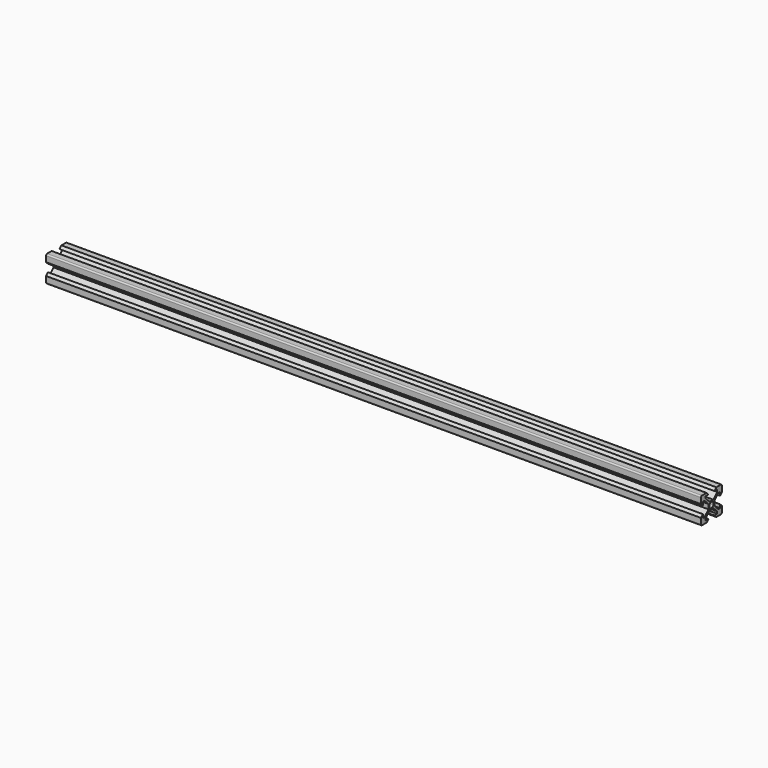
from build123d import *

# Parameters (mm, degrees)
F1_DEPTH = 500


# Not quite as in the source:
# - ends of sketch curves that miss each other by under 0.0002 mm in the source are joined


with BuildPart() as f1:
    # F0 (on Right) → F1 (new body)
    with BuildSketch(Plane.YZ):
        with BuildLine():
            Line((8.2, -10), (9, -10))
            ThreePointArc((9, -10), (9.7071067812, -9.7071067812), (10, -9))
            Line((10, -9), (10, -8.2))
            Line((10, -8.2), (8.2, -8.2))
            Line((8.2, -8.2), (8.2, -10))
        make_face()
        Polygon((5.4993398282, -8.2), (7.1393398282, -8.2), (5.4993398282, -6.56), align=None)
        Polygon((6.56, -5.4993398282), (8.2, -7.1393398282), (8.2, -5.4993398282), align=None)
        with BuildLine():
            Line((8.2, 10), (8.2, 8.2))
            Line((8.2, 8.2), (10, 8.2))
            Line((10, 8.2), (10, 9))
            ThreePointArc((10, 9), (9.7071067812, 9.7071067812), (9, 10))
            Line((9, 10), (8.2, 10))
        make_face()
        Polygon((8.2, 7.1393398282), (6.56, 5.4993398282), (8.2, 5.4993398282), align=None)
        Polygon((5.4993398282, 8.2), (5.4993398282, 6.56), (7.1393398282, 8.2), align=None)
        with BuildLine():
            Line((-9.9999004684, 8.2000055944), (-8.1999004684, 8.2000055944))
            Line((-8.1999004684, 8.2000055944), (-8.1999004684, 10.0000055944))
            Line((-8.1999004684, 10.0000055944), (-8.9999004684, 10.0000055944))
            ThreePointArc((-8.9999004684, 10.0000055944), (-9.7070072496, 9.7071123756), (-9.9999004684, 9.0000055944))
            Line((-9.9999004684, 9.0000055944), (-9.9999004684, 8.2000055944))
        make_face()
        Polygon((-7.1392402967, 8.2000055944), (-5.4992402967, 6.5600055944), (-5.4992402967, 8.2000055944), align=None)
        Polygon((-8.1999004684, 5.4993454226), (-6.5599004684, 5.4993454226), (-8.1999004684, 7.1393454226), align=None)
        with BuildLine():
            Line((-8.1999004684, -9.9999944056), (-8.1999004684, -8.1999944056))
            Line((-8.1999004684, -8.1999944056), (-9.9999004684, -8.1999944056))
            Line((-9.9999004684, -8.1999944056), (-9.9999004684, -8.9999944056))
            ThreePointArc((-9.9999004684, -8.9999944056), (-9.7070072496, -9.7071011868), (-8.9999004684, -9.9999944056))
            Line((-8.9999004684, -9.9999944056), (-8.1999004684, -9.9999944056))
        make_face()
        Polygon((-8.1999004684, -7.1393342338), (-6.5599004684, -5.4993342338), (-8.1999004684, -5.4993342338), align=None)
        Polygon((-5.4992402967, -8.1999944056), (-5.4992402967, -6.5599944056), (-7.1392402967, -8.1999944056), align=None)
        with BuildLine():
            Line((1.9173232366, -0.8566630648), (2.84, -1.7793398282))
            Line((2.84, -1.7793398282), (2.84, 0))
            Line((2.84, 0), (2.1, 0))
            ThreePointArc((2.1, 0), (2.0538231176, -0.4379618723), (1.9173232366, -0.8566630648))
        make_face()
        with BuildLine():
            Line((0, -2.84), (1.7793398282, -2.84))
            Line((1.7793398282, -2.84), (0.8566630648, -1.9173232366))
            ThreePointArc((0.8566630648, -1.9173232366), (0.4379618723, -2.0538231176), (0, -2.1))
            Line((0, -2.1), (0, -2.84))
        make_face()
        with BuildLine():
            Line((-1.7792402967, -2.8399944056), (9.95316e-05, -2.8399944056))
            Line((9.95316e-05, -2.8399944056), (0, -2.1))
            ThreePointArc((0, -2.1), (-0.4378623408, -2.0538175232), (-0.8565635332, -1.9173176422))
            Line((-0.8565635332, -1.9173176422), (-1.7792402967, -2.8399944056))
        make_face()
        Polygon((4.64, -10), (8.2, -10), (8.2, -8.2), (7.1393398282, -8.2), (5.4993398282, -8.2), (2.84, -8.2), align=None)
        Polygon((8.2, -8.2), (10, -8.2), (10, -4.64), (8.2, -2.84), (8.2, -5.4993398282), (8.2, -7.1393398282), align=None)
        with BuildLine():
            ThreePointArc((0, 2.1), (0.4379618723, 2.0538231176), (0.8566630648, 1.9173232366))
            Line((0.8566630648, 1.9173232366), (1.7793398282, 2.84))
            Line((1.7793398282, 2.84), (0, 2.84))
            Line((0, 2.84), (0, 2.1))
        make_face()
        with BuildLine():
            Line((2.1, 0), (2.84, 0))
            Line((2.84, 0), (2.84, 1.7793398282))
            Line((2.84, 1.7793398282), (1.9173232366, 0.8566630648))
            ThreePointArc((1.9173232366, 0.8566630648), (2.0538231176, 0.4379618723), (2.1, 0))
        make_face()
        with BuildLine():
            ThreePointArc((-0.8565635332, 1.917328831), (-0.4378623408, 2.053828712), (9.95316e-05, 2.1000055944))
            Line((9.95316e-05, 2.1000055944), (0, 2.84))
            Line((0, 2.84), (-1.7792402967, 2.8400055944))
            Line((-1.7792402967, 2.8400055944), (-0.8565635332, 1.917328831))
        make_face()
        Polygon((8.2, 8.2), (8.2, 7.1393398282), (8.2, 5.4993398282), (8.2, 2.84), (10, 4.64), (10, 8.2), align=None)
        Polygon((7.1393398282, 8.2), (8.2, 8.2), (8.2, 10), (4.64, 10), (2.84, 8.2), (5.4993398282, 8.2), align=None)
        with BuildLine():
            Line((-2.8399004684, 1.7793454226), (-2.8399004684, 5.5944e-06))
            Line((-2.8399004684, 5.5944e-06), (-2.0999004684, 5.5944e-06))
            ThreePointArc((-2.0999004684, 5.5944e-06), (-2.053723586, 0.4379674667), (-1.917223705, 0.8566686592))
            Line((-1.917223705, 0.8566686592), (-2.8399004684, 1.7793454226))
        make_face()
        Polygon((-8.1999004684, 10.0000055944), (-8.1999004684, 8.2000055944), (-7.1392402967, 8.2000055944), (-5.4992402967, 8.2000055944), (-2.8399004684, 8.2000055944), (-4.6399004684, 10.0000055944), align=None)
        Polygon((-8.1999004684, 5.4993454226), (-8.1999004684, 7.1393454226), (-8.1999004684, 8.2000055944), (-9.9999004684, 8.2000055944), (-9.9999004684, 4.6400055944), (-8.1999004684, 2.8400055944), align=None)
        with BuildLine():
            Line((-2.8399004684, 5.5944e-06), (-2.8399004684, -1.7793342338))
            Line((-2.8399004684, -1.7793342338), (-1.917223705, -0.8566574704))
            ThreePointArc((-1.917223705, -0.8566574704), (-2.053723586, -0.4379562779), (-2.0999004684, 5.5944e-06))
            Line((-2.0999004684, 5.5944e-06), (-2.8399004684, 5.5944e-06))
        make_face()
        Polygon((-9.9999004684, -8.1999944056), (-8.1999004684, -8.1999944056), (-8.1999004684, -7.1393342338), (-8.1999004684, -5.4993342338), (-8.1999004684, -2.8399944056), (-9.9999004684, -4.6399944056), align=None)
        Polygon((-5.4992402967, -8.1999944056), (-7.1392402967, -8.1999944056), (-8.1999004684, -8.1999944056), (-8.1999004684, -9.9999944056), (-4.6399004684, -9.9999944056), (-2.8399004684, -8.1999944056), align=None)
        with BuildLine():
            Line((-2.8399004684, -1.7793342338), (-1.7792402967, -2.8399944056))
            Line((-1.7792402967, -2.8399944056), (-0.8565635332, -1.9173176422))
            ThreePointArc((-0.8565635332, -1.9173176422), (-1.4848247089, -1.4849186461), (-1.917223705, -0.8566574704))
            Line((-1.917223705, -0.8566574704), (-2.8399004684, -1.7793342338))
        make_face()
        Polygon((-4.4695703825, -5.5303244915), (-1.7792402967, -2.8399944056), (-2.8399004684, -1.7793342338), (-5.5302305543, -4.4696643197), (-6.5599004684, -5.4993342338), (-8.1999004684, -7.1393342338), (-8.1999004684, -8.1999944056), (-7.1392402967, -8.1999944056), (-5.4992402967, -6.5599944056), align=None)
        with BuildLine():
            Line((7.1393398282, -8.2), (8.2, -8.2))
            Line((8.2, -8.2), (8.2, -7.1393398282))
            Line((8.2, -7.1393398282), (6.56, -5.4993398282))
            Line((6.56, -5.4993398282), (5.5303300859, -4.4696699141))
            Line((5.5303300859, -4.4696699141), (2.84, -1.7793398282))
            Line((2.84, -1.7793398282), (1.9173232366, -0.8566630648))
            ThreePointArc((1.9173232366, -0.8566630648), (1.4849242405, -1.4849242405), (0.8566630648, -1.9173232366))
            Line((0.8566630648, -1.9173232366), (1.7793398282, -2.84))
            Line((1.7793398282, -2.84), (4.4696699141, -5.5303300859))
            Line((4.4696699141, -5.5303300859), (5.4993398282, -6.56))
            Line((5.4993398282, -6.56), (7.1393398282, -8.2))
        make_face()
        with BuildLine():
            Line((1.9173232366, 0.8566630648), (2.84, 1.7793398282))
            Line((2.84, 1.7793398282), (5.5303300859, 4.4696699141))
            Line((5.5303300859, 4.4696699141), (6.56, 5.4993398282))
            Line((6.56, 5.4993398282), (8.2, 7.1393398282))
            Line((8.2, 7.1393398282), (8.2, 8.2))
            Line((8.2, 8.2), (7.1393398282, 8.2))
            Line((7.1393398282, 8.2), (5.4993398282, 6.56))
            Line((5.4993398282, 6.56), (4.4696699141, 5.5303300859))
            Line((4.4696699141, 5.5303300859), (1.7793398282, 2.84))
            Line((1.7793398282, 2.84), (0.8566630648, 1.9173232366))
            ThreePointArc((0.8566630648, 1.9173232366), (1.4849242405, 1.4849242405), (1.9173232366, 0.8566630648))
        make_face()
        with BuildLine():
            Line((-5.5302305543, 4.4696755085), (-2.8399004684, 1.7793454226))
            Line((-2.8399004684, 1.7793454226), (-1.917223705, 0.8566686592))
            ThreePointArc((-1.917223705, 0.8566686592), (-1.4848247089, 1.4849298349), (-0.8565635332, 1.917328831))
            Line((-0.8565635332, 1.917328831), (-1.7792402967, 2.8400055944))
            Line((-1.7792402967, 2.8400055944), (-4.4695703825, 5.5303356803))
            Line((-4.4695703825, 5.5303356803), (-5.4992402967, 6.5600055944))
            Line((-5.4992402967, 6.5600055944), (-7.1392402967, 8.2000055944))
            Line((-7.1392402967, 8.2000055944), (-8.1999004684, 8.2000055944))
            Line((-8.1999004684, 8.2000055944), (-8.1999004684, 7.1393454226))
            Line((-8.1999004684, 7.1393454226), (-6.5599004684, 5.4993454226))
            Line((-6.5599004684, 5.4993454226), (-5.5302305543, 4.4696755085))
        make_face()
    extrude(amount=F1_DEPTH)


solid = f1.part
